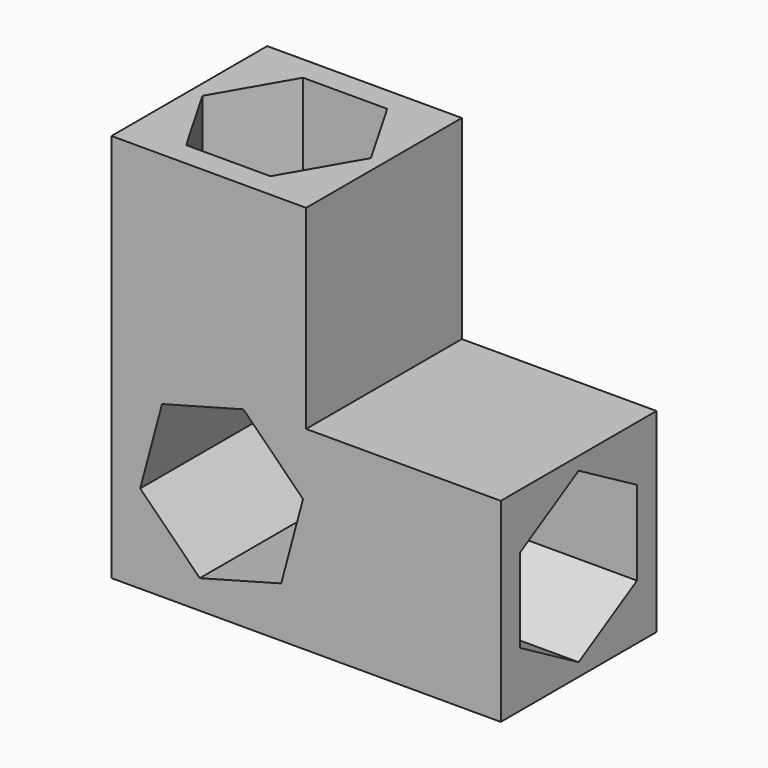
from build123d import *

# Parameters (mm, degrees)
F1_DEPTH = 12.7
F3_DEPTH = 9.525
F5_DEPTH = 9.525


# Not quite as in the source:
# - a feature names something its author has since deleted; it is built from what else it names


with BuildPart() as f1:
    # F0 (on Front) → F1 (new body)
    with BuildSketch(Plane.XZ):
        Polygon((-2.1617002284, 25.4), (-14.8617002284, 25.4), (-14.8617002284, 0), (10.5382997716, 0), (10.5382997716, 12.7), (-2.1617002284, 12.7), align=None)
        Polygon((-6.2541817694, 12.4960834256), (-2.3656168028, 8.6075184589), (-3.7889303648, 3.2956399302), (-9.1008088936, 1.8723263681), (-12.9893738602, 5.7608913348), (-11.5660602982, 11.0727698635), align=None, mode=Mode.SUBTRACT)
    extrude(amount=F1_DEPTH)

    # F2 (on face) → F3 (cut)
    with BuildSketch(Plane.XY.offset(25.4)):
        Polygon((-5.7620695714, -11.1125), (-3.0124389143, -6.35), (-5.7620695714, -1.5875), (-11.2613308854, -1.5875), (-14.0109615424, -6.35), (-11.2613308854, -11.1125), align=None)
    extrude(amount=-F3_DEPTH, mode=Mode.SUBTRACT)

    # F4 (on face) → F5 (cut)
    with BuildSketch(Plane.YZ.offset(10.5382997716)):
        Polygon((-6.35, 0.850738686), (-1.5875, 3.600369343), (-1.5875, 9.099630657), (-6.35, 11.849261314), (-11.1125, 9.099630657), (-11.1125, 3.600369343), align=None)
    extrude(amount=-F5_DEPTH, mode=Mode.SUBTRACT)


solid = f1.part
